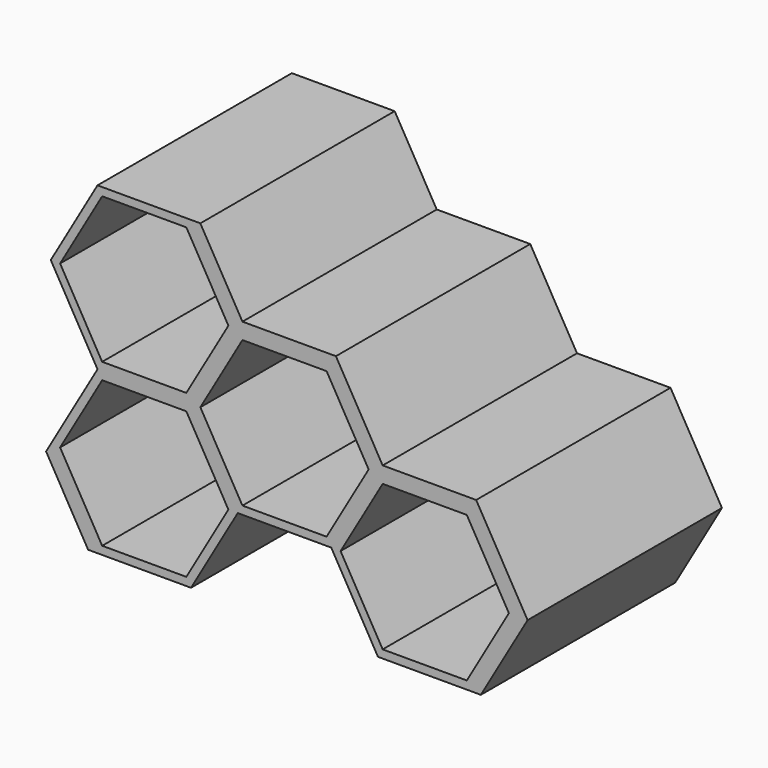
from build123d import *

# Parameters (mm, degrees)
F1_DEPTH = 12.7
F2_DEPTH = 95.25


# Not quite as in the source:
# - a feature names something its author has since deleted; it is built from what else it names


with BuildPart() as f1:
    # F0 (on Front) → F1 (new body)
    with BuildSketch(Plane.XZ):
        Polygon((87.3760877519, 66.7924993012), (50.7143456583, 66.7924993012), (32.3834746116, 35.0424993012), (50.7143456583, 3.2924993012), (87.3760877518, 3.2924993011), (105.7069587986, 35.0424993011), align=None)
        Polygon((52.547432763, 6.4674993012), (36.0496488209, 35.0424993012), (52.547432763, 63.6174993012), (85.5430006472, 63.6174993011), (102.0407845893, 35.0424993011), (85.5430006472, 6.4674993011), align=None, mode=Mode.SUBTRACT)
        Polygon((50.7143456583, 130.2924993012), (32.3834746116, 98.5424993012), (50.7143456583, 66.7924993012), (87.3760877519, 66.7924993012), (105.7069587986, 98.5424993012), (87.3760877519, 130.2924993012), align=None)
        Polygon((52.547432763, 69.9674993012), (36.0496488209, 98.5424993012), (52.547432763, 127.1174993012), (85.5430006472, 127.1174993012), (102.0407845893, 98.5424993012), (85.5430006472, 69.9674993012), align=None, mode=Mode.SUBTRACT)
        Polygon((160.699571939, 66.7924993012), (142.3687008922, 35.0424993012), (160.6995719389, 3.2924993011), (197.3613140325, 3.2924993011), (215.6921850793, 35.0424993012), (197.3613140325, 66.7924993012), align=None)
        Polygon((162.5326590436, 6.4674993012), (146.0348751015, 35.0424993012), (162.5326590436, 63.6174993012), (195.5282269278, 63.6174993012), (212.0260108699, 35.0424993012), (195.5282269278, 6.4674993012), align=None, mode=Mode.SUBTRACT)
        Polygon((105.7069587986, 98.5424993012), (87.3760877519, 66.7924993012), (105.7069587986, 35.0424993011), (142.3687008922, 35.0424993011), (160.699571939, 66.7924993012), (142.3687008922, 98.5424993012), align=None)
        Polygon((107.5400459033, 38.2174993012), (91.0422619612, 66.7924993012), (107.5400459033, 95.3674993012), (140.5356137875, 95.3674993012), (157.0333977296, 66.7924993012), (140.5356137875, 38.2174993012), align=None, mode=Mode.SUBTRACT)
        Polygon((52.547432763, 127.1174993012), (36.0496488209, 98.5424993012), (52.547432763, 69.9674993012), (85.5430006472, 69.9674993012), (102.0407845893, 98.5424993012), (85.5430006472, 127.1174993012), align=None)
        Polygon((52.547432763, 63.6174993012), (36.0496488209, 35.0424993012), (52.547432763, 6.4674993012), (85.5430006472, 6.4674993011), (102.0407845893, 35.0424993011), (85.5430006472, 63.6174993011), align=None)
        Polygon((162.5326590436, 63.6174993012), (146.0348751015, 35.0424993012), (162.5326590436, 6.4674993012), (195.5282269278, 6.4674993012), (212.0260108699, 35.0424993012), (195.5282269278, 63.6174993012), align=None)
        Polygon((107.5400459033, 95.3674993012), (91.0422619612, 66.7924993012), (107.5400459033, 38.2174993012), (140.5356137875, 38.2174993012), (157.0333977296, 66.7924993012), (140.5356137875, 95.3674993012), align=None)
    extrude(amount=F1_DEPTH)

    # F0 (on Front) → F2 (join)
    with BuildSketch(Plane.XZ):
        Polygon((50.7143456583, 130.2924993012), (32.3834746116, 98.5424993012), (50.7143456583, 66.7924993012), (87.3760877519, 66.7924993012), (105.7069587986, 98.5424993012), (87.3760877519, 130.2924993012), align=None)
        Polygon((52.547432763, 69.9674993012), (36.0496488209, 98.5424993012), (52.547432763, 127.1174993012), (85.5430006472, 127.1174993012), (102.0407845893, 98.5424993012), (85.5430006472, 69.9674993012), align=None, mode=Mode.SUBTRACT)
        Polygon((87.3760877519, 66.7924993012), (50.7143456583, 66.7924993012), (32.3834746116, 35.0424993012), (50.7143456583, 3.2924993012), (87.3760877518, 3.2924993011), (105.7069587986, 35.0424993011), align=None)
        Polygon((52.547432763, 6.4674993012), (36.0496488209, 35.0424993012), (52.547432763, 63.6174993012), (85.5430006472, 63.6174993011), (102.0407845893, 35.0424993011), (85.5430006472, 6.4674993011), align=None, mode=Mode.SUBTRACT)
        Polygon((105.7069587986, 98.5424993012), (87.3760877519, 66.7924993012), (105.7069587986, 35.0424993011), (142.3687008922, 35.0424993011), (160.699571939, 66.7924993012), (142.3687008922, 98.5424993012), align=None)
        Polygon((107.5400459033, 38.2174993012), (91.0422619612, 66.7924993012), (107.5400459033, 95.3674993012), (140.5356137875, 95.3674993012), (157.0333977296, 66.7924993012), (140.5356137875, 38.2174993012), align=None, mode=Mode.SUBTRACT)
        Polygon((160.699571939, 66.7924993012), (142.3687008922, 35.0424993012), (160.6995719389, 3.2924993011), (197.3613140325, 3.2924993011), (215.6921850793, 35.0424993012), (197.3613140325, 66.7924993012), align=None)
        Polygon((162.5326590436, 6.4674993012), (146.0348751015, 35.0424993012), (162.5326590436, 63.6174993012), (195.5282269278, 63.6174993012), (212.0260108699, 35.0424993012), (195.5282269278, 6.4674993012), align=None, mode=Mode.SUBTRACT)
        Polygon((91.0422619612, 130.2924993012), (87.3760877519, 130.2924993012), (105.7069587986, 98.5424993012), (142.3687008922, 98.5424993012), (160.699571939, 66.7924993012), (197.3613140325, 66.7924993012), (215.6921850793, 35.0424993012), (197.3613140325, 3.2924993012), (201.0274882418, 3.2924993011), (219.3583592886, 35.0424993012), (199.1944011372, 69.9674993012), (162.5326590436, 69.9674993012), (144.2017879969, 101.7174993012), (107.5400459033, 101.7174993012), align=None)
        Polygon((50.7143456583, 3.2924993012), (32.3834746116, 35.0424993012), (30.5503875069, 31.8674993012), (47.048171449, 3.2924993012), align=None)
    extrude(amount=F2_DEPTH)


solid = f1.part
